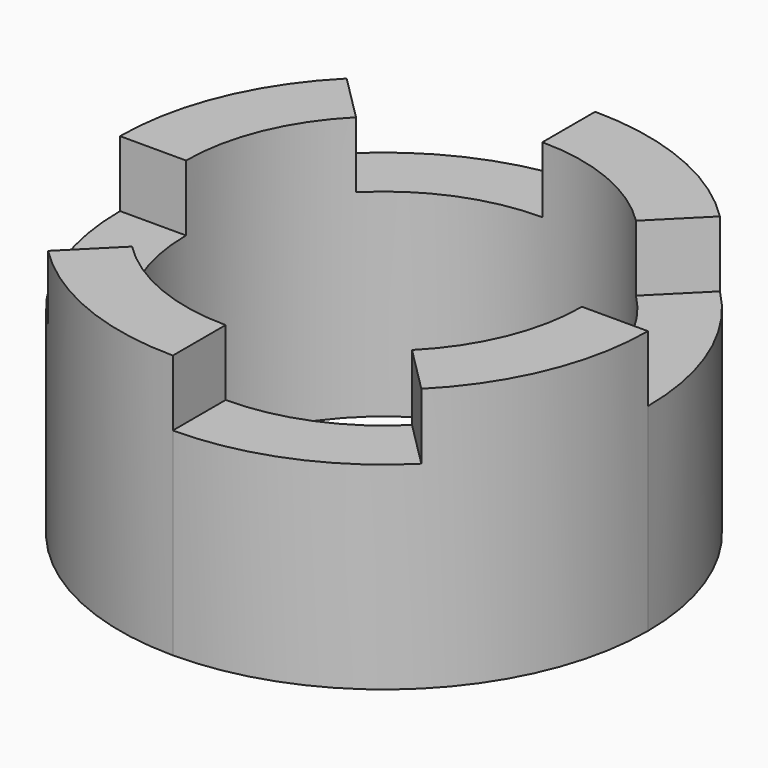
from build123d import *

# Parameters (mm, degrees)
F0_W     = 5.08
F0_H     = 3.175
F1_DEPTH = 25.4
F2_R     = 12.69999
F3_R     = 9.525
F4_DEPTH = 12.701
F6_DEPTH = 3.175


# Not quite as in the source:
# - a fillet or chamfer is up to 0.001 mm smaller than in the source, because OpenCascade refuses the exact size
# - ends of sketch curves that miss each other by under 0.0002 mm in the source are joined


with BuildPart() as f1:
    # F0 (on Front) → F1 (new body)
    with BuildSketch(Plane.XZ):
        Polygon((25.4, 0), (25.4, 12.7), (20.32, 12.7), (20.32, 9.525), (15.24, 9.525), (15.24, 12.7), (10.16, 12.7), (10.16, 9.525), (5.08, 9.525), (5.08, 12.7), (0, 12.7), (0, 0), align=None)
        with Locations((17.78, 11.1125)):
            Rectangle(F0_W, F0_H)
        with Locations((7.62, 11.1125)):
            Rectangle(F0_W, F0_H)
    extrude(amount=F1_DEPTH)

    # F2 (radius 12.7 in the source; OpenCascade refuses exactly that, so slightly less here)
    f2_edges = [f1.edges().sort_by_distance(p)[0] for p in [
        (0, -25.4, 6.35),
        (25.4, -25.4, 6.35),
        (25.4, 0, 6.35),
        (0, 0, 6.35),
    ]]
    fillet(f2_edges, radius=F2_R)

    # F3 (on face) → F4 (cut, through all)
    with BuildSketch(Plane.XY.offset(12.7)):
        with Locations((12.7, -12.7)):
            Circle(F3_R)
    extrude(amount=-F4_DEPTH, mode=Mode.SUBTRACT)

    # F5 (on face) → F6 (cut)
    with BuildSketch(Plane.XY.offset(12.7)):
        with BuildLine():
            ThreePointArc((19.4351920908, -19.4351920908), (21.4999525472, -16.3450596933), (22.225, -12.7))
            ThreePointArc((22.225, -12.7), (21.4999525472, -9.0549403067), (19.4351920908, -5.9648079092))
            ThreePointArc((19.4351920908, -5.9648079092), (16.3450596933, -3.9000474528), (12.7, -3.175))
            ThreePointArc((12.7, -3.175), (9.0549403067, -3.9000474528), (5.9648079092, -5.9648079092))
            ThreePointArc((5.9648079092, -5.9648079092), (3.9000474528, -9.0549403067), (3.175, -12.7))
            ThreePointArc((3.175, -12.7), (3.9000474528, -16.3450596933), (5.9648079092, -19.4351920908))
            ThreePointArc((5.9648079092, -19.4351920908), (9.0549403067, -21.4999525472), (12.7, -22.225))
            ThreePointArc((12.7, -22.225), (16.3450596933, -21.4999525472), (19.4351920908, -19.4351920908))
        make_face()
        with BuildLine():
            ThreePointArc((12.69999, 0), (7.8399142358, -0.9667291759), (3.71974095, -3.71974095))
            Line((3.71974095, -3.71974095), (5.9648079092, -5.9648079092))
            ThreePointArc((5.9648079092, -5.9648079092), (9.0549403067, -3.9000474528), (12.7, -3.175))
            Line((12.7, -3.175), (12.69999, 0))
        make_face()
        with BuildLine():
            ThreePointArc((25.4, -12.69999), (24.4332708241, -7.8399142358), (21.68025905, -3.71974095))
            Line((21.68025905, -3.71974095), (19.4351920908, -5.9648079092))
            ThreePointArc((19.4351920908, -5.9648079092), (21.4999525472, -9.0549403067), (22.225, -12.7))
            Line((22.225, -12.7), (25.4, -12.69999))
        make_face()
        with BuildLine():
            Line((3.175, -12.7), (0, -12.7))
            ThreePointArc((0, -12.7), (0.9667291759, -17.5600857642), (3.71974095, -21.68025905))
            Line((3.71974095, -21.68025905), (5.9648079092, -19.4351920908))
            ThreePointArc((5.9648079092, -19.4351920908), (3.9000474528, -16.3450596933), (3.175, -12.7))
        make_face()
        with BuildLine():
            Line((12.7, -22.225), (12.7, -25.4))
            ThreePointArc((12.7, -25.4), (17.5600857642, -24.4332708241), (21.68025905, -21.68025905))
            Line((21.68025905, -21.68025905), (19.4351920908, -19.4351920908))
            ThreePointArc((19.4351920908, -19.4351920908), (16.3450596933, -21.4999525472), (12.7, -22.225))
        make_face()
    extrude(amount=-F6_DEPTH, mode=Mode.SUBTRACT)


solid = f1.part
